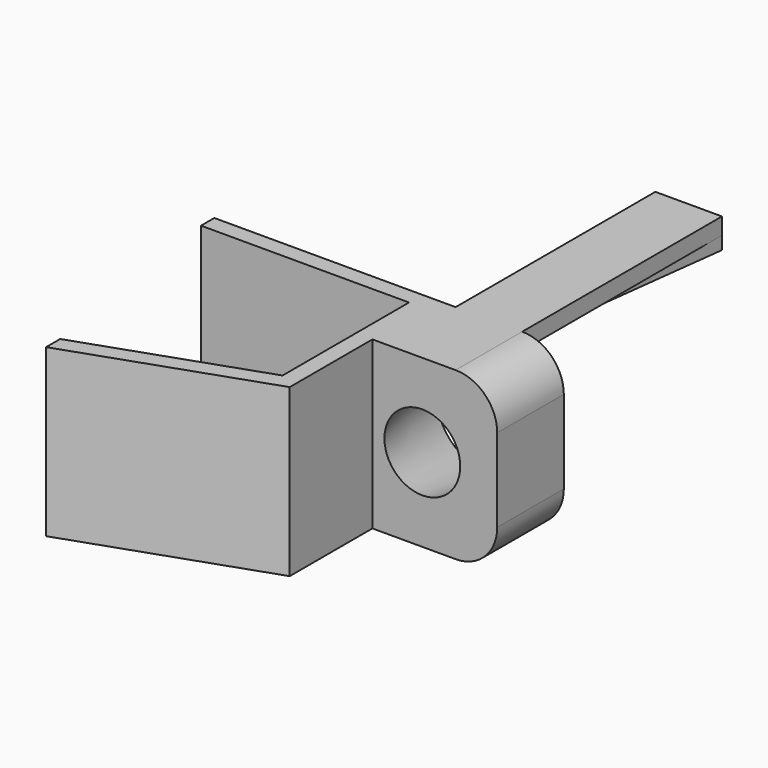
from build123d import *

# Parameters (mm, degrees)
F1_DEPTH               = 20
F2_R                   = 6.315
F3_DEPTH               = 10
F3_TAPER               = 10
F4_R                   = 5
F5_W                   = 8
F5_H                   = 2
F6_DEPTH               = 30
F8_DEPTH               = 30
DRAFT_F8_DRAFTED_ANGLE = 2.5


# Not quite as in the source:
# - an extrude with a draft is written as a straight extrude whose walls are then drafted


with BuildPart() as f1:
    # F0 (on Top) → F1 (new body)
    with BuildSketch(Plane.XY):
        Polygon((-61.5762866481, 4.9875803861), (-61.5762866481, 2.9875803861), (-36.5762866481, 2.9875803861), (-36.5762866481, -16.0124196139), (-57.5038306415, -23.2546203382), (-57.5038306415, -25.3709927201), (-34.5762866481, -17.4366705766), (-34.5762866481, -5.0124196139), (-19.5762866481, -5.0124196139), (-19.5762866481, 4.9875803861), align=None)
    extrude(amount=F1_DEPTH)

    # F2 (on face) → F3 (cut)
    with BuildSketch(Plane(origin=(0, 4.9875803861, 0), x_dir=(-1, 0, 0), z_dir=(0, 1, 0))):
        with Locations((28.5762866481, 10)):
            Circle(F2_R)
    extrude(amount=-F3_DEPTH, taper=F3_TAPER, mode=Mode.SUBTRACT)

    # F4
    f4_edges = [f1.edges().sort_by_distance(p)[0] for p in [
        (-19.576287, -0.01242, 20),
        (-19.576287, -0.01242, 0),
    ]]
    fillet(f4_edges, radius=F4_R)

    # F5 (on face) → F6 (join)
    with BuildSketch(Plane(origin=(0, 4.9875803861, 0), x_dir=(-1, 0, 0), z_dir=(0, 1, 0))):
        with Locations((28.5762866481, 19)):
            Rectangle(F5_W, F5_H)
    extrude(amount=F6_DEPTH)


with BuildPart() as f8_drafted:
    # F7 (on face) → F8 (new body)
    with BuildSketch(Plane(origin=(0, 34.9875803861, 0), x_dir=(-1, 0, 0), z_dir=(0, 1, 0))):
        with BuildLine():
            Line((24.5762866481, 20), (24.5762866481, 16.4336301386))
            ThreePointArc((24.5762866481, 16.4336301386), (28.5762866481, 17.026790883), (32.5762866481, 16.4336301386))
            Line((32.5762866481, 16.4336301386), (32.5762866481, 20))
            Line((32.5762866481, 20), (24.5762866481, 20))
        make_face()
    extrude(amount=-F8_DEPTH)

    # draft_F8_drafted
    draft_f8_drafted_walls = [f8_drafted.faces().sort_by_distance(p)[0] for p in [
        (-28.5762866481, 14.9875803861, 17.026790883),
        (-32.5762866481, 14.9875803861, 18.2168150693),
        (-28.5762866481, 14.9875803861, 20),
        (-24.5762866481, 14.9875803861, 18.2168150693),
    ]]
    draft(draft_f8_drafted_walls, neutral_plane=Plane(origin=(0, 34.9875803861, 0), x_dir=(-1, 0, 0), z_dir=(0, -1, 0)), angle=DRAFT_F8_DRAFTED_ANGLE)


with BuildPart() as f1_1:
    add(f1.part)

    # join_F8_drafted: union F8_drafted
    add(f8_drafted.part)


solid = f1_1.part
